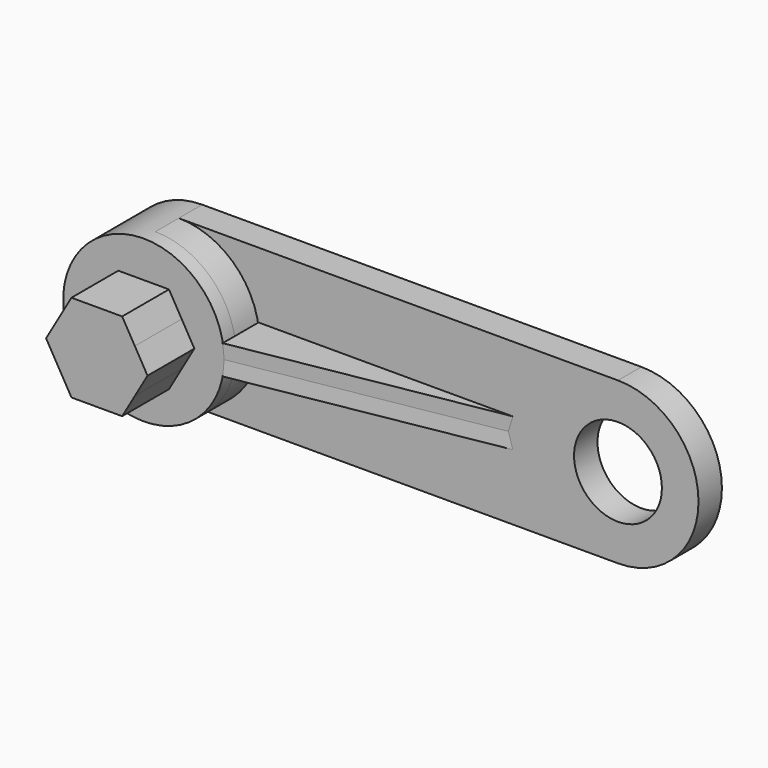
from build123d import *

# Parameters (mm, degrees)
F0_R      = 3
F1_DEPTH  = 2
F2_R      = 3
F3_DEPTH  = 2
F4_R      = 5.5
F4_R_2    = 3
F5_DEPTH  = 1
F7_DEPTH  = 4
F10_DEPTH = 1
F10_TAPER = -3


with BuildPart() as f1:
    # F0 (on Front) → F1 (new body)
    with BuildSketch(Plane.XZ):
        with BuildLine():
            Line((15, 5.5), (-15, 5.5))
            ThreePointArc((-15, 5.5), (-20.5, 0), (-15, -5.5))
            Line((-15, -5.5), (15, -5.5))
            ThreePointArc((15, -5.5), (20.5, 0), (15, 5.5))
        make_face()
        with Locations((-15, 0)):
            Circle(F0_R, mode=Mode.SUBTRACT)
        with Locations((15, 0)):
            Circle(F0_R, mode=Mode.SUBTRACT)
    extrude(amount=F1_DEPTH)

    # F2 (on face) → F3 (join)
    with BuildSketch(Plane.XZ.offset(2)):
        with BuildLine():
            ThreePointArc((-15, -5.5), (-11.110913, -3.889087), (-9.5, 0))
            ThreePointArc((-9.5, 0), (-11.110913, 3.889087), (-15, 5.5))
            ThreePointArc((-15, 5.5), (-20.5, 0), (-15, -5.5))
        make_face()
        with Locations((-15, 0)):
            Circle(F2_R, mode=Mode.SUBTRACT)
    extrude(amount=F3_DEPTH)

    # F4 (on face) → F5 (join)
    with BuildSketch(Plane.XZ.offset(4)):
        with Locations((-15, 0)):
            Circle(F4_R)
        with Locations((-15, 0)):
            Circle(F4_R_2, mode=Mode.SUBTRACT)
        with Locations((-15, 0)):
            Circle(F4_R_2)
    extrude(amount=F5_DEPTH)

    # F6 (on face) → F7 (join)
    with BuildSketch(Plane.XZ.offset(5)):
        with BuildLine():
            Line((-13.267949, -3), (-12.401924, -1.5))
            ThreePointArc((-12.401924, -1.5), (-13.5, -2.598076), (-15, -3))
            Line((-15, -3), (-13.267949, -3))
        make_face()
        with BuildLine():
            ThreePointArc((-12.401924, 1.5), (-12.102223, 0.776457), (-12, 0))
            ThreePointArc((-12, 0), (-12.102223, -0.776457), (-12.401924, -1.5))
            Line((-12.401924, -1.5), (-11.535898, 0))
            Line((-11.535898, 0), (-12.401924, 1.5))
        make_face()
        with BuildLine():
            ThreePointArc((-15, 3), (-13.5, 2.598076), (-12.401924, 1.5))
            Line((-12.401924, 1.5), (-13.267949, 3))
            Line((-13.267949, 3), (-15, 3))
        make_face()
        with BuildLine():
            ThreePointArc((-17.598076, -1.5), (-18, 0), (-17.598076, 1.5))
            Line((-17.598076, 1.5), (-18.464102, 0))
            Line((-18.464102, 0), (-17.598076, -1.5))
        make_face()
        with BuildLine():
            Line((-16.732051, -3), (-15, -3))
            ThreePointArc((-15, -3), (-16.5, -2.598076), (-17.598076, -1.5))
            Line((-17.598076, -1.5), (-16.732051, -3))
        make_face()
        with BuildLine():
            ThreePointArc((-12.401924, -1.5), (-12.102223, -0.776457), (-12, 0))
            ThreePointArc((-12, 0), (-12.102223, 0.776457), (-12.401924, 1.5))
            ThreePointArc((-12.401924, 1.5), (-13.5, 2.598076), (-15, 3))
            ThreePointArc((-15, 3), (-16.5, 2.598076), (-17.598076, 1.5))
            ThreePointArc((-17.598076, 1.5), (-18, 0), (-17.598076, -1.5))
            ThreePointArc((-17.598076, -1.5), (-16.5, -2.598076), (-15, -3))
            ThreePointArc((-15, -3), (-13.5, -2.598076), (-12.401924, -1.5))
        make_face()
        with BuildLine():
            ThreePointArc((-17.598076, 1.5), (-16.5, 2.598076), (-15, 3))
            Line((-15, 3), (-16.732051, 3))
            Line((-16.732051, 3), (-17.598076, 1.5))
        make_face()
    extrude(amount=F7_DEPTH)

    # F9 (on offset) → F10 (join, symmetric)
    with BuildSketch(Plane(origin=(0, 0, 0), x_dir=(1, 0, 0), z_dir=(0, 0, -1))):
        Polygon((7.513845, 2), (-9.5, 5), (-9.5, 2), align=None)
    extrude(amount=F10_DEPTH, both=True, taper=F10_TAPER)


solid = f1.part
